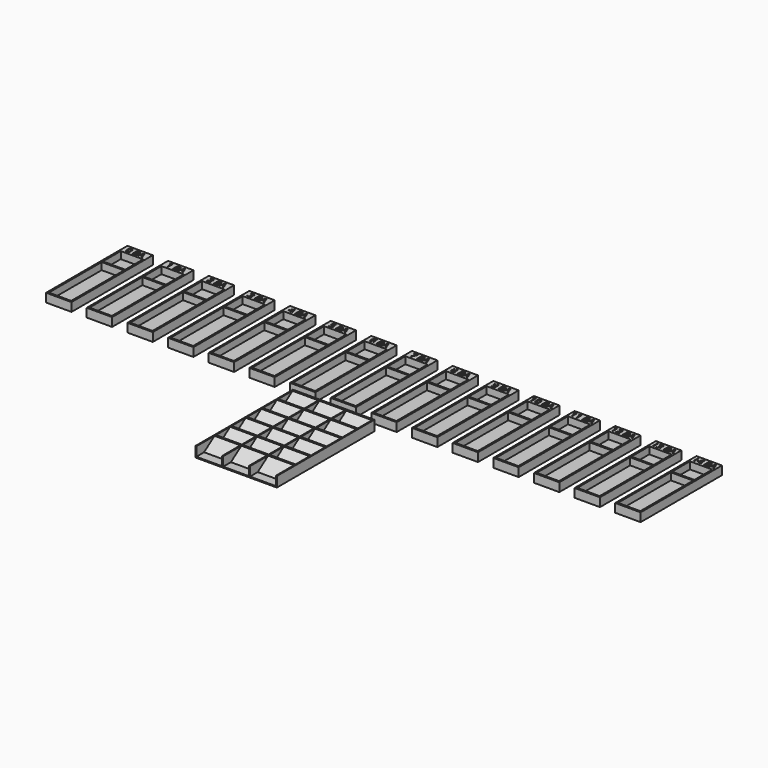
from build123d import *

# Parameters (mm, degrees)
F0_W         = 25
F0_H         = 100
F0_W_2       = 22
F0_H_2       = 22
F2_DEPTH     = 7
F1_W         = 25
F1_H         = 100
F3_DEPTH     = 1.5
F4_TEXT_SIZE = 8.3333333333
F5_TEXT_SIZE = 8.3333333333
F6_TEXT_SIZE = 8.3333333333
F7_TEXT_SIZE = 8.3333333333
F8_TEXT_SIZE = 8.3333333333
F9_TEXT_SIZE = 8.3333333333
F10_DEPTH    = 2
F11_W        = 1
F11_H        = 120
F11_W_2      = 25.4
F12_DEPTH    = 1
F13_DEPTH    = 10
F15_DEPTH    = 78.2


# Not quite as in the source:
# - Text() gives the source's letters only with a copy of the font that has no kerning and outlines rounded to 1/6400 em; it was checked with that copy


with BuildPart() as f2:
    # F0 (on Top) → F2 (new body)
    with BuildSketch(Plane.XY):
        with Locations((43.0518667399, 16.2181752287)):
            Rectangle(F0_W, F0_H)
        Polygon((32.0518667399, 32.7181752287), (42.3018667399, 32.7181752287), (43.8018667399, 32.7181752287), (54.0518667399, 32.7181752287), (54.0518667399, -32.2818247713), (43.8018667399, -32.2818247713), (42.3018667399, -32.2818247713), (32.0518667399, -32.2818247713), align=None, mode=Mode.SUBTRACT)
        with Locations((43.0518667399, 45.2181752287)):
            Rectangle(F0_W_2, F0_H_2, mode=Mode.SUBTRACT)
    extrude(amount=F2_DEPTH)

    # F1 (on Top) → F3 (join)
    with BuildSketch(Plane.XY):
        with Locations((43.0518667399, 16.2181752287)):
            Rectangle(F1_W, F1_H)
    extrude(amount=-F3_DEPTH)


with BuildPart() as f2b:
    # F0 (on Top) → F2, piece 2 (new body)
    with BuildSketch(Plane.XY):
        with Locations((83.0518667399, 16.2181752287)):
            Rectangle(F0_W, F0_H)
        Polygon((72.0518667399, -32.2818247713), (72.0518667399, 32.7181752287), (82.3018667399, 32.7181752287), (83.8018667399, 32.7181752287), (94.0518667399, 32.7181752287), (94.0518667399, -32.2818247713), (83.8018667399, -32.2818247713), (82.3018667399, -32.2818247713), align=None, mode=Mode.SUBTRACT)
        with Locations((83.0518667399, 45.2181752287)):
            Rectangle(F0_W_2, F0_H_2, mode=Mode.SUBTRACT)
    extrude(amount=F2_DEPTH)

    # F1 (on Top) → F3, piece 2 (join)
    with BuildSketch(Plane.XY):
        with Locations((83.0518667399, 16.2181752287)):
            Rectangle(F1_W, F1_H)
    extrude(amount=-F3_DEPTH)


with BuildPart() as f2c:
    # F0 (on Top) → F2, piece 3 (new body)
    with BuildSketch(Plane.XY):
        with Locations((123.0518667399, 16.2181752287)):
            Rectangle(F0_W, F0_H)
        Polygon((112.0518667399, -32.2818247713), (112.0518667399, 32.7181752287), (122.3018667399, 32.7181752287), (123.8018667399, 32.7181752287), (134.0518667399, 32.7181752287), (134.0518667399, -32.2818247713), (123.8018667399, -32.2818247713), (122.3018667399, -32.2818247713), align=None, mode=Mode.SUBTRACT)
        with Locations((123.0518667399, 45.2181752287)):
            Rectangle(F0_W_2, F0_H_2, mode=Mode.SUBTRACT)
    extrude(amount=F2_DEPTH)

    # F1 (on Top) → F3, piece 3 (join)
    with BuildSketch(Plane.XY):
        with Locations((123.0518667399, 16.2181752287)):
            Rectangle(F1_W, F1_H)
    extrude(amount=-F3_DEPTH)


with BuildPart() as f2d:
    # F0 (on Top) → F2, piece 4 (new body)
    with BuildSketch(Plane.XY):
        with Locations((163.0518667399, 16.2181752287)):
            Rectangle(F0_W, F0_H)
        Polygon((152.0518667399, -32.2818247713), (152.0518667399, 32.7181752287), (162.3018667399, 32.7181752287), (163.8018667399, 32.7181752287), (174.0518667399, 32.7181752287), (174.0518667399, -32.2818247713), (163.8018667399, -32.2818247713), (162.3018667399, -32.2818247713), align=None, mode=Mode.SUBTRACT)
        with Locations((163.0518667399, 45.2181752287)):
            Rectangle(F0_W_2, F0_H_2, mode=Mode.SUBTRACT)
    extrude(amount=F2_DEPTH)

    # F1 (on Top) → F3, piece 4 (join)
    with BuildSketch(Plane.XY):
        with Locations((163.0518667399, 16.2181752287)):
            Rectangle(F1_W, F1_H)
    extrude(amount=-F3_DEPTH)


with BuildPart() as f2e:
    # F0 (on Top) → F2, piece 5 (new body)
    with BuildSketch(Plane.XY):
        with Locations((203.0518667399, 16.2181752287)):
            Rectangle(F0_W, F0_H)
        Polygon((192.0518667399, -32.2818247713), (192.0518667399, 32.7181752287), (202.3018667399, 32.7181752287), (203.8018667399, 32.7181752287), (214.0518667399, 32.7181752287), (214.0518667399, -32.2818247713), (203.8018667399, -32.2818247713), (202.3018667399, -32.2818247713), align=None, mode=Mode.SUBTRACT)
        with Locations((203.0518667399, 45.2181752287)):
            Rectangle(F0_W_2, F0_H_2, mode=Mode.SUBTRACT)
    extrude(amount=F2_DEPTH)

    # F1 (on Top) → F3, piece 5 (join)
    with BuildSketch(Plane.XY):
        with Locations((203.0518667399, 16.2181752287)):
            Rectangle(F1_W, F1_H)
    extrude(amount=-F3_DEPTH)


with BuildPart() as f2f:
    # F0 (on Top) → F2, piece 6 (new body)
    with BuildSketch(Plane.XY):
        with Locations((243.0518667399, 16.2181752287)):
            Rectangle(F0_W, F0_H)
        Polygon((232.0518667399, -32.2818247713), (232.0518667399, 32.7181752287), (242.3018667399, 32.7181752287), (243.8018667399, 32.7181752287), (254.0518667399, 32.7181752287), (254.0518667399, -32.2818247713), (243.8018667399, -32.2818247713), (242.3018667399, -32.2818247713), align=None, mode=Mode.SUBTRACT)
        with Locations((243.0518667399, 45.2181752287)):
            Rectangle(F0_W_2, F0_H_2, mode=Mode.SUBTRACT)
    extrude(amount=F2_DEPTH)

    # F1 (on Top) → F3, piece 6 (join)
    with BuildSketch(Plane.XY):
        with Locations((243.0518667399, 16.2181752287)):
            Rectangle(F1_W, F1_H)
    extrude(amount=-F3_DEPTH)


with BuildPart() as f2g:
    # F0 (on Top) → F2, piece 7 (new body)
    with BuildSketch(Plane.XY):
        with Locations((283.0518667399, 16.2181752287)):
            Rectangle(F0_W, F0_H)
        Polygon((272.0518667399, -32.2818247713), (272.0518667399, 32.7181752287), (282.3018667399, 32.7181752287), (283.8018667399, 32.7181752287), (294.0518667399, 32.7181752287), (294.0518667399, -32.2818247713), (283.8018667399, -32.2818247713), (282.3018667399, -32.2818247713), align=None, mode=Mode.SUBTRACT)
        with Locations((283.0518667399, 45.2181752287)):
            Rectangle(F0_W_2, F0_H_2, mode=Mode.SUBTRACT)
    extrude(amount=F2_DEPTH)

    # F1 (on Top) → F3, piece 7 (join)
    with BuildSketch(Plane.XY):
        with Locations((283.0518667399, 16.2181752287)):
            Rectangle(F1_W, F1_H)
    extrude(amount=-F3_DEPTH)


with BuildPart() as f2h:
    # F0 (on Top) → F2, piece 8 (new body)
    with BuildSketch(Plane.XY):
        with Locations((323.0518667399, 16.2181752287)):
            Rectangle(F0_W, F0_H)
        Polygon((312.0518667399, -32.2818247713), (312.0518667399, 32.7181752287), (322.3018667399, 32.7181752287), (323.8018667399, 32.7181752287), (334.0518667399, 32.7181752287), (334.0518667399, -32.2818247713), (323.8018667399, -32.2818247713), (322.3018667399, -32.2818247713), align=None, mode=Mode.SUBTRACT)
        with Locations((323.0518667399, 45.2181752287)):
            Rectangle(F0_W_2, F0_H_2, mode=Mode.SUBTRACT)
    extrude(amount=F2_DEPTH)

    # F1 (on Top) → F3, piece 8 (join)
    with BuildSketch(Plane.XY):
        with Locations((323.0518667399, 16.2181752287)):
            Rectangle(F1_W, F1_H)
    extrude(amount=-F3_DEPTH)


with BuildPart() as f2i:
    # F0 (on Top) → F2, piece 9 (new body)
    with BuildSketch(Plane.XY):
        with Locations((363.0518667399, 16.2181752287)):
            Rectangle(F0_W, F0_H)
        Polygon((352.0518667399, -32.2818247713), (352.0518667399, 32.7181752287), (362.3018667399, 32.7181752287), (363.8018667399, 32.7181752287), (374.0518667399, 32.7181752287), (374.0518667399, -32.2818247713), (363.8018667399, -32.2818247713), (362.3018667399, -32.2818247713), align=None, mode=Mode.SUBTRACT)
        with Locations((363.0518667399, 45.2181752287)):
            Rectangle(F0_W_2, F0_H_2, mode=Mode.SUBTRACT)
    extrude(amount=F2_DEPTH)

    # F1 (on Top) → F3, piece 9 (join)
    with BuildSketch(Plane.XY):
        with Locations((363.0518667399, 16.2181752287)):
            Rectangle(F1_W, F1_H)
    extrude(amount=-F3_DEPTH)


with BuildPart() as f2j:
    # F0 (on Top) → F2, piece 10 (new body)
    with BuildSketch(Plane.XY):
        with Locations((403.0518667399, 16.2181752287)):
            Rectangle(F0_W, F0_H)
        Polygon((392.0518667399, -32.2818247713), (392.0518667399, 32.7181752287), (402.3018667399, 32.7181752287), (403.8018667399, 32.7181752287), (414.0518667399, 32.7181752287), (414.0518667399, -32.2818247713), (403.8018667399, -32.2818247713), (402.3018667399, -32.2818247713), align=None, mode=Mode.SUBTRACT)
        with Locations((403.0518667399, 45.2181752287)):
            Rectangle(F0_W_2, F0_H_2, mode=Mode.SUBTRACT)
    extrude(amount=F2_DEPTH)

    # F1 (on Top) → F3, piece 10 (join)
    with BuildSketch(Plane.XY):
        with Locations((403.0518667399, 16.2181752287)):
            Rectangle(F1_W, F1_H)
    extrude(amount=-F3_DEPTH)


with BuildPart() as f2k:
    # F0 (on Top) → F2, piece 11 (new body)
    with BuildSketch(Plane.XY):
        with Locations((443.0518667399, 16.2181752287)):
            Rectangle(F0_W, F0_H)
        Polygon((432.0518667399, -32.2818247713), (432.0518667399, 32.7181752287), (442.3018667399, 32.7181752287), (443.8018667399, 32.7181752287), (454.0518667399, 32.7181752287), (454.0518667399, -32.2818247713), (443.8018667399, -32.2818247713), (442.3018667399, -32.2818247713), align=None, mode=Mode.SUBTRACT)
        with Locations((443.0518667399, 45.2181752287)):
            Rectangle(F0_W_2, F0_H_2, mode=Mode.SUBTRACT)
    extrude(amount=F2_DEPTH)

    # F1 (on Top) → F3, piece 11 (join)
    with BuildSketch(Plane.XY):
        with Locations((443.0518667399, 16.2181752287)):
            Rectangle(F1_W, F1_H)
    extrude(amount=-F3_DEPTH)


with BuildPart() as f2l:
    # F0 (on Top) → F2, piece 12 (new body)
    with BuildSketch(Plane.XY):
        with Locations((483.0518667399, 16.2181752287)):
            Rectangle(F0_W, F0_H)
        Polygon((472.0518667399, -32.2818247713), (472.0518667399, 32.7181752287), (482.3018667399, 32.7181752287), (483.8018667399, 32.7181752287), (494.0518667399, 32.7181752287), (494.0518667399, -32.2818247713), (483.8018667399, -32.2818247713), (482.3018667399, -32.2818247713), align=None, mode=Mode.SUBTRACT)
        with Locations((483.0518667399, 45.2181752287)):
            Rectangle(F0_W_2, F0_H_2, mode=Mode.SUBTRACT)
    extrude(amount=F2_DEPTH)

    # F1 (on Top) → F3, piece 12 (join)
    with BuildSketch(Plane.XY):
        with Locations((483.0518667399, 16.2181752287)):
            Rectangle(F1_W, F1_H)
    extrude(amount=-F3_DEPTH)


with BuildPart() as f2m:
    # F0 (on Top) → F2, piece 13 (new body)
    with BuildSketch(Plane.XY):
        with Locations((523.0518667399, 16.2181752287)):
            Rectangle(F0_W, F0_H)
        Polygon((512.0518667399, -32.2818247713), (512.0518667399, 32.7181752287), (522.3018667399, 32.7181752287), (523.8018667399, 32.7181752287), (534.0518667399, 32.7181752287), (534.0518667399, -32.2818247713), (523.8018667399, -32.2818247713), (522.3018667399, -32.2818247713), align=None, mode=Mode.SUBTRACT)
        with Locations((523.0518667399, 45.2181752287)):
            Rectangle(F0_W_2, F0_H_2, mode=Mode.SUBTRACT)
    extrude(amount=F2_DEPTH)

    # F1 (on Top) → F3, piece 13 (join)
    with BuildSketch(Plane.XY):
        with Locations((523.0518667399, 16.2181752287)):
            Rectangle(F1_W, F1_H)
    extrude(amount=-F3_DEPTH)


with BuildPart() as f2n:
    # F0 (on Top) → F2, piece 14 (new body)
    with BuildSketch(Plane.XY):
        with Locations((563.0518667399, 16.2181752287)):
            Rectangle(F0_W, F0_H)
        Polygon((552.0518667399, -32.2818247713), (552.0518667399, 32.7181752287), (562.3018667399, 32.7181752287), (563.8018667399, 32.7181752287), (574.0518667399, 32.7181752287), (574.0518667399, -32.2818247713), (563.8018667399, -32.2818247713), (562.3018667399, -32.2818247713), align=None, mode=Mode.SUBTRACT)
        with Locations((563.0518667399, 45.2181752287)):
            Rectangle(F0_W_2, F0_H_2, mode=Mode.SUBTRACT)
    extrude(amount=F2_DEPTH)

    # F1 (on Top) → F3, piece 14 (join)
    with BuildSketch(Plane.XY):
        with Locations((563.0518667399, 16.2181752287)):
            Rectangle(F1_W, F1_H)
    extrude(amount=-F3_DEPTH)


with BuildPart() as f2o:
    # F0 (on Top) → F2, piece 15 (new body)
    with BuildSketch(Plane.XY):
        with Locations((603.0518667399, 16.2181752287)):
            Rectangle(F0_W, F0_H)
        Polygon((592.0518667399, -32.2818247713), (592.0518667399, 32.7181752287), (602.3018667399, 32.7181752287), (603.8018667399, 32.7181752287), (614.0518667399, 32.7181752287), (614.0518667399, -32.2818247713), (603.8018667399, -32.2818247713), (602.3018667399, -32.2818247713), align=None, mode=Mode.SUBTRACT)
        with Locations((603.0518667399, 45.2181752287)):
            Rectangle(F0_W_2, F0_H_2, mode=Mode.SUBTRACT)
    extrude(amount=F2_DEPTH)

    # F1 (on Top) → F3, piece 15 (join)
    with BuildSketch(Plane.XY):
        with Locations((603.0518667399, 16.2181752287)):
            Rectangle(F1_W, F1_H)
    extrude(amount=-F3_DEPTH)


with BuildPart() as f10_tool:
    # F4 (on face) + F5 (on face) + F6 (on face) + F7 (on face) + F8 (on face) + F9 (on face) → F10 (new body)
    with BuildSketch(Plane.XY.offset(7)):
        with Locations((33.9802521565, 58.2181752287)):
            Text('0 BA', F4_TEXT_SIZE, font='Open Sans', text_align=(TextAlign.LEFT, TextAlign.BOTTOM))
    with BuildSketch(Plane.XY.offset(7)):
        with Locations((73.9802521565, 58.2181752287)):
            Text('1 BA', F5_TEXT_SIZE, font='Open Sans', text_align=(TextAlign.LEFT, TextAlign.BOTTOM))
    with BuildSketch(Plane.XY.offset(7)):
        with Locations((113.9802521565, 58.2181752287)):
            Text('2 BA', F6_TEXT_SIZE, font='Open Sans', text_align=(TextAlign.LEFT, TextAlign.BOTTOM))
    with BuildSketch(Plane.XY.offset(7)):
        with Locations((153.9802521565, 58.2181752287)):
            Text('3 BA', F7_TEXT_SIZE, font='Open Sans', text_align=(TextAlign.LEFT, TextAlign.BOTTOM))
    with BuildSketch(Plane.XY.offset(7)):
        with Locations((193.9802521565, 58.2181752287)):
            Text('4 BA', F8_TEXT_SIZE, font='Open Sans', text_align=(TextAlign.LEFT, TextAlign.BOTTOM))
    with BuildSketch(Plane.XY.offset(7)):
        with Locations((233.9802521565, 58.2181752287)):
            Text('5 BA', F9_TEXT_SIZE, font='Open Sans', text_align=(TextAlign.LEFT, TextAlign.BOTTOM))
        with Locations((273.9802521565, 58.2181752287)):
            Text('6 BA', F9_TEXT_SIZE, font='Open Sans', text_align=(TextAlign.LEFT, TextAlign.BOTTOM))
        with Locations((313.9802521565, 58.2181752287)):
            Text('7 BA', F9_TEXT_SIZE, font='Open Sans', text_align=(TextAlign.LEFT, TextAlign.BOTTOM))
        with Locations((353.9802521565, 58.2181752287)):
            Text('8 BA', F9_TEXT_SIZE, font='Open Sans', text_align=(TextAlign.LEFT, TextAlign.BOTTOM))
        with Locations((393.9802521565, 58.2181752287)):
            Text('9 BA', F9_TEXT_SIZE, font='Open Sans', text_align=(TextAlign.LEFT, TextAlign.BOTTOM))
        with Locations((431.5980906982, 58.2181752287)):
            Text('10 BA', F9_TEXT_SIZE, font='Open Sans', text_align=(TextAlign.LEFT, TextAlign.BOTTOM))
        with Locations((471.5980906982, 58.2181752287)):
            Text('11 BA', F9_TEXT_SIZE, font='Open Sans', text_align=(TextAlign.LEFT, TextAlign.BOTTOM))
        with Locations((511.5980906982, 58.2181752287)):
            Text('12 BA', F9_TEXT_SIZE, font='Open Sans', text_align=(TextAlign.LEFT, TextAlign.BOTTOM))
        with Locations((551.5980906982, 58.2181752287)):
            Text('13 BA', F9_TEXT_SIZE, font='Open Sans', text_align=(TextAlign.LEFT, TextAlign.BOTTOM))
        with Locations((591.5980906982, 58.2181752287)):
            Text('14 BA', F9_TEXT_SIZE, font='Open Sans', text_align=(TextAlign.LEFT, TextAlign.BOTTOM))
    extrude(amount=-F10_DEPTH)


with BuildPart() as f2_1:
    add(f2.part)

    # F10: cut by f10_tool
    add(f10_tool.part, mode=Mode.SUBTRACT)


with BuildPart() as f2b_1:
    add(f2b.part)

    # F10: cut by f10_tool
    add(f10_tool.part, mode=Mode.SUBTRACT)


with BuildPart() as f2c_1:
    add(f2c.part)

    # F10: cut by f10_tool
    add(f10_tool.part, mode=Mode.SUBTRACT)


with BuildPart() as f2d_1:
    add(f2d.part)

    # F10: cut by f10_tool
    add(f10_tool.part, mode=Mode.SUBTRACT)


with BuildPart() as f2e_1:
    add(f2e.part)

    # F10: cut by f10_tool
    add(f10_tool.part, mode=Mode.SUBTRACT)


with BuildPart() as f2f_1:
    add(f2f.part)

    # F10: cut by f10_tool
    add(f10_tool.part, mode=Mode.SUBTRACT)


with BuildPart() as f2g_1:
    add(f2g.part)

    # F10: cut by f10_tool
    add(f10_tool.part, mode=Mode.SUBTRACT)


with BuildPart() as f2h_1:
    add(f2h.part)

    # F10: cut by f10_tool
    add(f10_tool.part, mode=Mode.SUBTRACT)


with BuildPart() as f2i_1:
    add(f2i.part)

    # F10: cut by f10_tool
    add(f10_tool.part, mode=Mode.SUBTRACT)


with BuildPart() as f2j_1:
    add(f2j.part)

    # F10: cut by f10_tool
    add(f10_tool.part, mode=Mode.SUBTRACT)


with BuildPart() as f2k_1:
    add(f2k.part)

    # F10: cut by f10_tool
    add(f10_tool.part, mode=Mode.SUBTRACT)


with BuildPart() as f2l_1:
    add(f2l.part)

    # F10: cut by f10_tool
    add(f10_tool.part, mode=Mode.SUBTRACT)


with BuildPart() as f2m_1:
    add(f2m.part)

    # F10: cut by f10_tool
    add(f10_tool.part, mode=Mode.SUBTRACT)


with BuildPart() as f2n_1:
    add(f2n.part)

    # F10: cut by f10_tool
    add(f10_tool.part, mode=Mode.SUBTRACT)


with BuildPart() as f2o_1:
    add(f2o.part)

    # F10: cut by f10_tool
    add(f10_tool.part, mode=Mode.SUBTRACT)


with BuildPart() as f12:
    # F11 (on Top) → F12 (new body)
    with BuildSketch(Plane.XY):
        with Locations((283.4692747477, -105.7018942032)):
            Rectangle(F11_W, F11_H)
        with Locations((296.6692747477, -105.7018942032)):
            Rectangle(F11_W_2, F11_H)
        with Locations((309.8692747477, -105.7018942032)):
            Rectangle(F11_W, F11_H)
        with Locations((323.0692747477, -105.7018942032)):
            Rectangle(F11_W_2, F11_H)
        with Locations((336.2692747477, -105.7018942032)):
            Rectangle(F11_W, F11_H)
        with Locations((349.4692747477, -105.7018942032)):
            Rectangle(F11_W_2, F11_H)
        with Locations((362.6692747477, -105.7018942032)):
            Rectangle(F11_W, F11_H)
    extrude(amount=F12_DEPTH)

    # F11 (on Top) → F13 (join)
    with BuildSketch(Plane.XY):
        with Locations((283.4692747477, -105.7018942032)):
            Rectangle(F11_W, F11_H)
        with Locations((309.8692747477, -105.7018942032)):
            Rectangle(F11_W, F11_H)
        with Locations((336.2692747477, -105.7018942032)):
            Rectangle(F11_W, F11_H)
        with Locations((362.6692747477, -105.7018942032)):
            Rectangle(F11_W, F11_H)
    extrude(amount=F13_DEPTH)

    # F14 (on face) → F15 (join, through all)
    with BuildSketch(Plane.YZ.offset(283.9692747477)):
        Polygon((-47.4453409989, 10), (-60.2986730595, 1), (-58.5552262639, 1), (-45.7018942032, 10), align=None)
        Polygon((-79.4765878114, 1), (-77.7331410158, 1), (-64.8798089551, 10), (-66.6232557507, 10), align=None)
        Polygon((-98.6545025632, 1), (-96.9110557676, 1), (-84.0577237069, 10), (-85.8011705025, 10), align=None)
        Polygon((-117.832417315, 1), (-116.0889705194, 1), (-103.2356384587, 10), (-104.9790852544, 10), align=None)
        Polygon((-137.0103320669, 1), (-135.2668852713, 1), (-122.4135532106, 10), (-124.1570000062, 10), align=None)
        Polygon((-156.1882468187, 1), (-154.4448000231, 1), (-141.5914679624, 10), (-143.334914758, 10), align=None)
    extrude(amount=F15_DEPTH)


solid = Compound([f2_1.part, f2b_1.part, f2c_1.part, f2d_1.part, f2e_1.part, f2f_1.part, f2g_1.part, f2h_1.part, f2i_1.part, f2j_1.part, f2k_1.part, f2l_1.part, f2m_1.part, f2n_1.part, f2o_1.part, f12.part])
